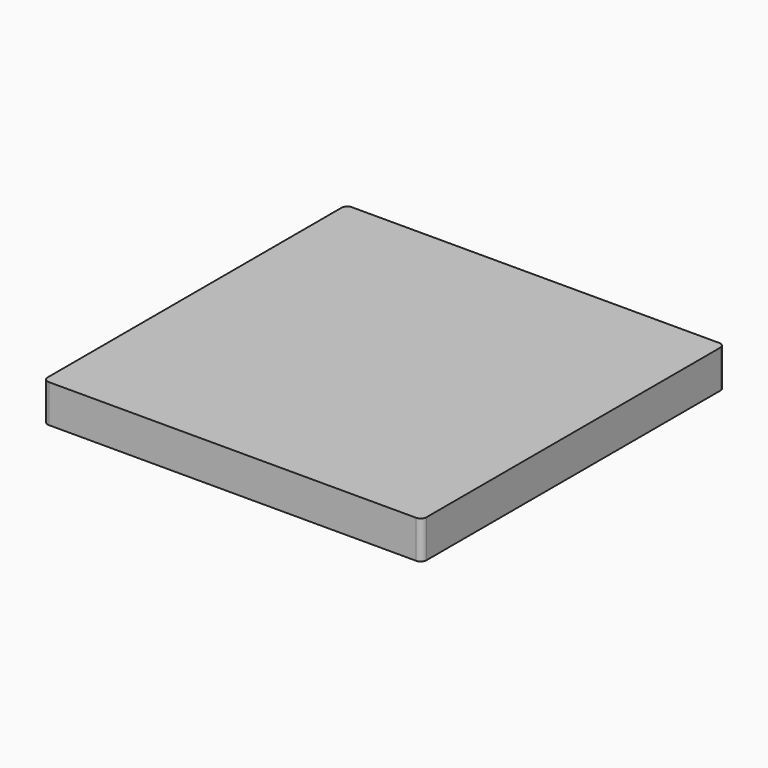
from build123d import *

# Parameters (mm, degrees)
F0_W     = 500
F0_H     = 500
F0_R     = 118.0247003556
F0_W_2   = 75
F0_H_2   = 75
F1_DEPTH = 50
F2_DEPTH = 40
F3_R     = 7.5


with BuildPart() as f1:
    # F0 (on Top) → F1 (new body)
    with BuildSketch(Plane.XY):
        Rectangle(F0_W, F0_H)
        Polygon((-191.2311762839, 43.6472680867), (-85.1058798965, 176.7241805792), (85.1058798965, 176.7241805792), (191.2311762839, 43.6472680867), (153.3554965244, -122.296927517), (0, -196.1490422978), (-153.3554965244, -122.296927517), align=None, mode=Mode.SUBTRACT)
        Polygon((85.1058798965, 176.7241805792), (-85.1058798965, 176.7241805792), (-191.2311762839, 43.6472680867), (-153.3554965244, -122.296927517), (0, -196.1490422978), (153.3554965244, -122.296927517), (191.2311762839, 43.6472680867), align=None)
        Circle(F0_R, mode=Mode.SUBTRACT)
        Circle(F0_R)
        Rectangle(F0_W_2, F0_H_2, mode=Mode.SUBTRACT)
        Rectangle(F0_W_2, F0_H_2)
    extrude(amount=F1_DEPTH)

    # F0 (on Top) → F2 (cut)
    with BuildSketch(Plane.XY):
        Polygon((85.1058798965, 176.7241805792), (-85.1058798965, 176.7241805792), (-191.2311762839, 43.6472680867), (-153.3554965244, -122.296927517), (0, -196.1490422978), (153.3554965244, -122.296927517), (191.2311762839, 43.6472680867), align=None)
        Circle(F0_R, mode=Mode.SUBTRACT)
        Rectangle(F0_W_2, F0_H_2)
    extrude(amount=F2_DEPTH, mode=Mode.SUBTRACT)

    # F3
    f3_edges = [f1.edges().sort_by_distance(p)[0] for p in [
        (250, -250, 25),
        (-250, -250, 25),
        (-250, 250, 25),
        (250, 250, 25),
        (0, -196.149042, 20),
        (-153.355497, -122.296928, 20),
        (153.355497, -122.296928, 20),
        (191.231176, 43.647268, 20),
        (85.10588, 176.724181, 20),
        (-85.10588, 176.724181, 20),
        (-191.231176, 43.647268, 20),
        (-37.5, -37.5, 20),
        (37.5, -37.5, 20),
        (37.5, 37.5, 20),
        (-37.5, 37.5, 20),
    ]]
    fillet(f3_edges, radius=F3_R)


solid = f1.part
